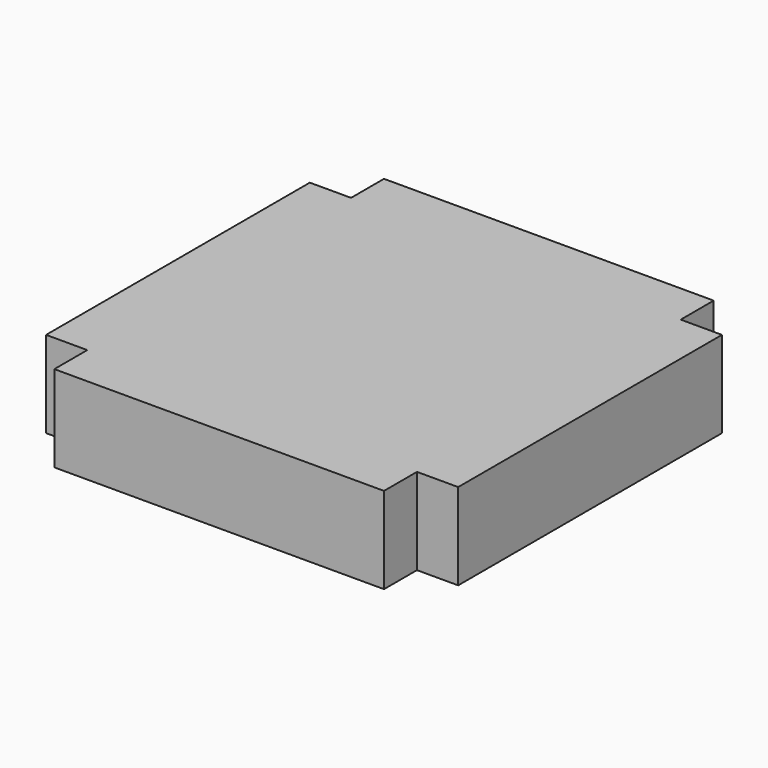
from build123d import *

# Parameters (mm, degrees)
F1_DEPTH = 20
F2_T     = -1
F3_R     = 24
F4_DEPTH = 19
F5_T     = -1
F7_DEPTH = 1


# Not quite as in the source:
# - a shell that OpenCascade refuses in one call is made with other operations: the cavity is built on its own and cut out


with BuildPart() as f1:
    # F0 (on Top) → F1 (new body)
    with BuildSketch(Plane.XY):
        Polygon((40, 50), (-40, 50), (-40, 40), (-50, 40), (-50, -40), (-40, -40), (-40, -50), (40, -50), (40, -40), (50, -40), (50, 40), (40, 40), align=None)
    extrude(amount=F1_DEPTH)

    # F2
    f2_openings = [f1.faces().sort_by_distance(p)[0] for p in [
        (0, 0, 20),
    ]]
    offset(amount=F2_T, openings=f2_openings, kind=Kind.INTERSECTION)

    # F3 (on face) → F4 (join)
    with BuildSketch(Plane.XY.offset(1)):
        Circle(F3_R)
    extrude(amount=F4_DEPTH)

    # F5: a shell. OpenCascade refuses it in one call, so the cavity is built on its own and cut out:
    # the body offset inwards by the wall thickness, plus a prism from it out through each open face.
    f5_core = offset(f1.part, amount=F5_T, kind=Kind.INTERSECTION, mode=Mode.PRIVATE)
    f5_exits = [f5_core.faces().sort_by_distance(p)[0] for p in [
        (0, 0, 19),
    ]]
    add(f5_core, mode=Mode.SUBTRACT)
    extrude(f5_exits, amount=-F5_T, mode=Mode.SUBTRACT)

    # F6 (on face) → F7 (join)
    with BuildSketch(Plane.XY.offset(20)):
        Polygon((-40, -50), (40, -50), (40, -40), (50, -40), (50, 40), (40, 40), (40, 50), (-40, 50), (-40, 40), (-50, 40), (-50, -40), (-40, -40), align=None)
    extrude(amount=F7_DEPTH)


solid = f1.part
